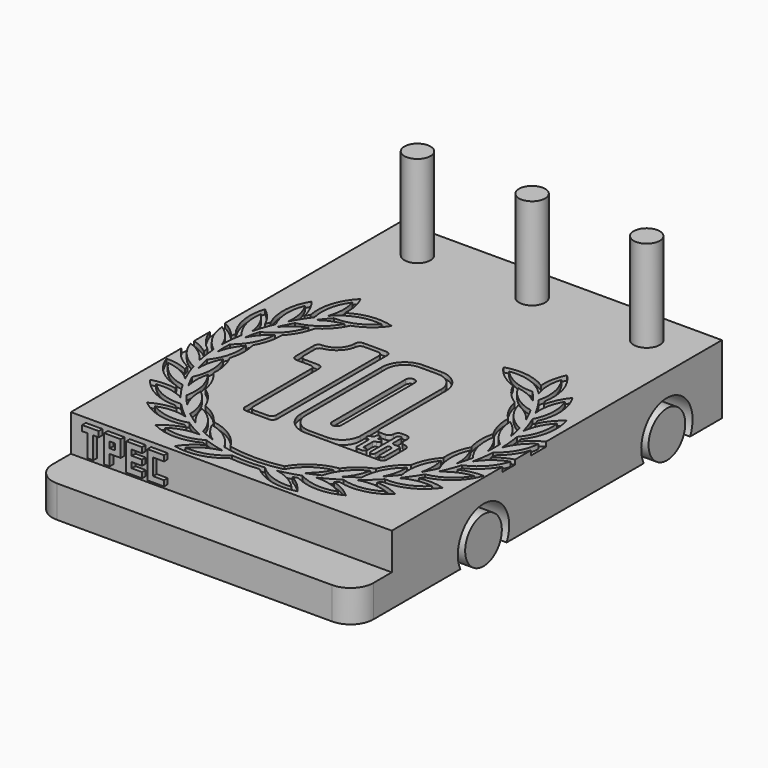
from build123d import *

# Parameters (mm, degrees)
F0_W           = 70
F0_H           = 100
F1_DEPTH       = 15
F2_W           = 70
F2_H           = 10
F3_DEPTH       = 8
F4_R           = 2.85
F5_DEPTH       = 20
F7_R           = 5
F8_DEPTH       = 35
F8_DEPTH_BACK  = 35
F10_DEPTH      = 25
F10_DEPTH_BACK = 25
F11_R          = 7
F11_R_2        = 5
F12_DEPTH      = 10
F13_R          = 7
F13_R_2        = 5
F14_DEPTH      = 10
F15_R          = 5
F16_W          = 1.2
F16_H          = 1.3280942544
F17_DEPTH      = 1
F19_DEPTH      = 1
F21_DEPTH      = 1
F23_DEPTH      = 1
F24_R          = 0.99999
F25_R          = 0.49999


# Not quite as in the source:
# - a fillet or chamfer is up to 0.001 mm smaller than in the source, because OpenCascade refuses the exact size
# - ends of sketch curves that miss each other by under 0.0002 mm in the source are joined


with BuildPart() as f1:
    # F0 (on Top) → F1 (new body)
    with BuildSketch(Plane.XY):
        Rectangle(F0_W, F0_H)
    extrude(amount=F1_DEPTH)

    # F2 (on face) → F3 (cut)
    with BuildSketch(Plane.XY.offset(15)):
        with Locations((0, -45)):
            Rectangle(F2_W, F2_H)
    extrude(amount=-F3_DEPTH, mode=Mode.SUBTRACT)

    # F4 (on face) → F5 (join)
    with BuildSketch(Plane.XY.offset(15)):
        with Locations((0, 42)):
            Circle(F4_R)
        with Locations((-25, 42)):
            Circle(F4_R)
        with Locations((25, 42)):
            Circle(F4_R)
    extrude(amount=F5_DEPTH)

    # F7 (on Right) → F8 (join, two sides)
    with BuildSketch(Plane.YZ) as f8_sk:
        with Locations((-15, 3)):
            Circle(F7_R)
        with Locations((35, 3)):
            Circle(F7_R)
    extrude(amount=F8_DEPTH)
    extrude(f8_sk.sketch, amount=-F8_DEPTH_BACK)

    # F9 (on Right) → F10 (cut, two sides)
    with BuildSketch(Plane.YZ) as f10_sk:
        with BuildLine():
            Line((-11, 0), (-19, 0))
            ThreePointArc((-19, 0), (-15, -2), (-11, 0))
        make_face()
        with BuildLine():
            Line((39, 0), (31, 0))
            ThreePointArc((31, 0), (35, -2), (39, 0))
        make_face()
    extrude(amount=-F10_DEPTH, mode=Mode.SUBTRACT)
    extrude(f10_sk.sketch, amount=F10_DEPTH_BACK, mode=Mode.SUBTRACT)

    # F11 (on face) → F12 (cut)
    with BuildSketch(Plane.YZ.offset(35)):
        with Locations((-15, 3)):
            Circle(F11_R)
        with Locations((-15, 3)):
            Circle(F11_R_2, mode=Mode.SUBTRACT)
        with Locations((35, 3)):
            Circle(F11_R)
        with Locations((35, 3)):
            Circle(F11_R_2, mode=Mode.SUBTRACT)
    extrude(amount=-F12_DEPTH, mode=Mode.SUBTRACT)

    # F13 (on face) → F14 (cut)
    with BuildSketch(Plane(origin=(-35, 0, 0), x_dir=(0, -1, 0), z_dir=(-1, 0, 0))):
        with Locations((15, 3)):
            Circle(F13_R)
        with Locations((15, 3)):
            Circle(F13_R_2, mode=Mode.SUBTRACT)
        with Locations((-35, 3)):
            Circle(F13_R)
        with Locations((-35, 3)):
            Circle(F13_R_2, mode=Mode.SUBTRACT)
    extrude(amount=-F14_DEPTH, mode=Mode.SUBTRACT)

    # F15
    f15_edges = [f1.edges().sort_by_distance(p)[0] for p in [
        (35, -50, 3.5),
        (-35, -50, 3.5),
    ]]
    fillet(f15_edges, radius=F15_R)

    # F16 (on face) → F17 (join)
    with BuildSketch(Plane.XZ.offset(40)):
        Polygon((-28.1147292094, 14), (-31.7147292094, 14), (-31.7147292094, 12.8), (-30.5147292094, 12.8), (-30.5147292094, 8), (-29.3147292094, 8), (-29.3147292094, 12.8), (-28.1147292094, 12.8), align=None)
        Polygon((-23.3147292094, 14), (-26.9147292094, 14), (-26.9147292094, 8), (-25.7147292094, 8), (-25.7147292094, 10.4), (-23.3147292094, 10.4), align=None)
        with Locations((-25.1147292094, 12.1359528728)):
            Rectangle(F16_W, F16_H, mode=Mode.SUBTRACT)
        Polygon((-18.6747292094, 14), (-22.1147292094, 14), (-22.1147292094, 8), (-18.6747292094, 8), (-18.6747292094, 9.2), (-20.9147292094, 9.2), (-20.9147292094, 10.4), (-18.6747292094, 10.4), (-18.6747292094, 11.6), (-20.9147292094, 11.6), (-20.9147292094, 12.8), (-18.6747292094, 12.8), align=None)
        Polygon((-13.8747292094, 12.8), (-13.8747292094, 14), (-17.4747292094, 14), (-17.4747292094, 8), (-13.8747292094, 8), (-13.8747292094, 9.2), (-16.2747292094, 9.2), (-16.2747292094, 12.8), align=None)
    extrude(amount=F17_DEPTH)

    # F18 (on face) → F19 (cut)
    with BuildSketch(Plane.XY.offset(15)):
        with BuildLine():
            ThreePointArc((21.3887258181, 17.7264092206), (16.9142472373, 19.3626016034), (12.1676058235, 18.953359167))
            ThreePointArc((12.1676058235, 18.953359167), (14.591215486, 16.340180418), (17.7231115659, 14.6390590482))
            ThreePointArc((17.7231115659, 14.6390590482), (19.4200221668, 12.0422463003), (21.7744615029, 10.0224548638))
            ThreePointArc((21.7744615029, 10.0224548638), (22.8267654259, 7.1043050239), (24.6519445841, 4.5959862493))
            ThreePointArc((24.6519445841, 4.5959862493), (25.0029118524, 1.5138175305), (26.2004349519, -1.3478044677))
            ThreePointArc((26.2004349519, -1.3478044677), (25.8311448292, -4.427831552), (26.3364530897, -7.4884859913))
            ThreePointArc((26.3364530897, -7.4884859913), (25.2668141021, -10.4003263836), (25.0526662245, -13.4950125909))
            ThreePointArc((25.0526662245, -13.4950125909), (23.3403428867, -16.0816882221), (22.4182836385, -19.0435708628))
            ThreePointArc((22.4182836385, -19.0435708628), (20.1555877448, -21.1656333801), (18.5753255788, -23.8350365945))
            ThreePointArc((18.5753255788, -23.8350365945), (15.8842396506, -25.3780850583), (13.7309669091, -27.6111006282))
            ThreePointArc((13.7309669091, -27.6111006282), (9.2041132945, -29.3610412569), (5.8709446294, -32.888743413))
            ThreePointArc((5.8709446294, -32.888743413), (0, -33.5), (-5.8709446294, -32.888743413))
            ThreePointArc((-5.8709446294, -32.888743413), (-9.2041132945, -29.3610412569), (-13.7309669091, -27.6111006282))
            ThreePointArc((-13.7309669091, -27.6111006282), (-15.8842396506, -25.3780850583), (-18.5753255788, -23.8350365945))
            ThreePointArc((-18.5753255788, -23.8350365945), (-20.1555877448, -21.1656333801), (-22.4182836385, -19.0435708628))
            ThreePointArc((-22.4182836385, -19.0435708628), (-23.3403428867, -16.0816882221), (-25.0526662245, -13.4950125909))
            ThreePointArc((-25.0526662245, -13.4950125909), (-25.2668141021, -10.4003263836), (-26.3364530897, -7.4884859913))
            ThreePointArc((-26.3364530897, -7.4884859913), (-25.8311448292, -4.427831552), (-26.2004349519, -1.3478044677))
            ThreePointArc((-26.2004349519, -1.3478044677), (-25.0029118524, 1.5138175305), (-24.6519445841, 4.5959862493))
            ThreePointArc((-24.6519445841, 4.5959862493), (-22.8267654259, 7.1043050239), (-21.7744615029, 10.0224548638))
            ThreePointArc((-21.7744615029, 10.0224548638), (-19.4200221668, 12.0422463003), (-17.7231115659, 14.6390590482))
            ThreePointArc((-17.7231115659, 14.6390590482), (-14.591215486, 16.340180418), (-12.1676058235, 18.953359167))
            ThreePointArc((-12.1676058235, 18.953359167), (-16.9142472373, 19.3626016034), (-21.3887258181, 17.7264092206))
            ThreePointArc((-21.3887258181, 17.7264092206), (-21.5697046499, 20.6456209174), (-22.5135920697, 23.4139465498))
            ThreePointArc((-22.5135920697, 23.4139465498), (-25.2629047542, 18.8188140189), (-25.5168178808, 13.4700299198))
            ThreePointArc((-25.5168178808, 13.4700299198), (-25.8263883801, 13.0346240116), (-26.1285301404, 12.5940305986))
            ThreePointArc((-26.1285301404, 12.5940305986), (-26.9914700696, 15.1700718344), (-28.4594423065, 17.4560533046))
            ThreePointArc((-28.4594423065, 17.4560533046), (-30.074936422, 12.350748027), (-29.088490785, 7.0875846987))
            ThreePointArc((-29.088490785, 7.0875846987), (-29.2893052588, 6.5925233429), (-29.4816949152, 6.0941274973))
            ThreePointArc((-29.4816949152, 6.0941274973), (-30.9154501797, 8.401723565), (-32.8710366422, 10.2875484131))
            ThreePointArc((-32.8710366422, 10.2875484131), (-33.2656204828, 4.9472987179), (-31.0919956218, 0.0534946578))
            ThreePointArc((-31.0919956218, 0.0534946578), (-31.1732281098, -0.4745332598), (-31.2454938862, -1.0038628891))
            ThreePointArc((-31.2454938862, -1.0038628891), (-32.9521784804, 0.735711305), (-35, 2.0568160339))
            Line((-35, 2.0568160339), (-35, -2.1009931114))
            ThreePointArc((-35, -2.1009931114), (-33.5847749975, -4.9377165589), (-31.4193229266, -7.2530305881))
            ThreePointArc((-31.4193229266, -7.2530305881), (-31.3765941644, -7.7855589458), (-31.3248401941, -8.3172860614))
            ThreePointArc((-31.3248401941, -8.3172860614), (-33.0705923516, -7.1776978407), (-35, -6.38795229))
            Line((-35, -6.38795229), (-35, -9.7772099505))
            ThreePointArc((-35, -9.7772099505), (-32.8954370333, -12.4993428364), (-30.0528264, -14.4380943719))
            ThreePointArc((-30.0528264, -14.4380943719), (-29.8884399062, -14.9464144281), (-29.7154562591, -15.4518734835))
            ThreePointArc((-29.7154562591, -15.4518734835), (-32.2970706727, -14.6057524582), (-35.0073216617, -14.4181535604))
            ThreePointArc((-35.0073216617, -14.4181535604), (-31.8769440834, -18.762655768), (-27.0661742232, -21.1143480451))
            ThreePointArc((-27.0661742232, -21.1143480451), (-26.7889921162, -21.571056134), (-26.5041043855, -22.0229977008))
            ThreePointArc((-26.5041043855, -22.0229977008), (-29.2112599855, -21.7950452331), (-31.8917190916, -22.2375299796))
            ThreePointArc((-31.8917190916, -22.2375299796), (-27.8438100865, -25.743010817), (-22.6203775882, -26.9218730442))
            ThreePointArc((-22.6203775882, -26.9218730442), (-22.2453428272, -27.3023479145), (-21.8639093842, -27.6764077058))
            ThreePointArc((-21.8639093842, -27.6764077058), (-24.5506627115, -28.0789127723), (-27.0568256903, -29.1276266959))
            ThreePointArc((-27.0568256903, -29.1276266959), (-22.3096090807, -31.6051047837), (-16.9551105424, -31.5475841932))
            ThreePointArc((-16.9551105424, -31.5475841932), (-16.5024413484, -31.8313143462), (-16.0450253688, -32.1073267018))
            ThreePointArc((-16.0450253688, -32.1073267018), (-18.566532856, -33.1185901502), (-20.7632918127, -34.7169968119))
            ThreePointArc((-20.7632918127, -34.7169968119), (-15.5726912747, -36.0329106651), (-10.3757890986, -34.7421082068))
            ThreePointArc((-10.3757890986, -34.7421082068), (-9.869888985, -34.9137976764), (-9.3611498826, -35.0768826988))
            ThreePointArc((-9.3611498826, -35.0768826988), (-11.5814764084, -36.6423870548), (-13.3504034991, -38.7043159377))
            ThreePointArc((-13.3504034991, -38.7043159377), (-7.9962456512, -38.7877243), (-3.2371061788, -36.3332274684))
            ThreePointArc((-3.2371061788, -36.3332274684), (0, -36.5), (3.2371061788, -36.3332274684))
            ThreePointArc((3.2371061788, -36.3332274684), (7.9962456512, -38.7877243), (13.3504034991, -38.7043159377))
            ThreePointArc((13.3504034991, -38.7043159377), (11.5814764084, -36.6423870548), (9.3611498826, -35.0768826988))
            ThreePointArc((9.3611498826, -35.0768826988), (9.869888985, -34.9137976764), (10.3757890986, -34.7421082068))
            ThreePointArc((10.3757890986, -34.7421082068), (15.5726912747, -36.0329106651), (20.7632918127, -34.7169968119))
            ThreePointArc((20.7632918127, -34.7169968119), (18.566532856, -33.1185901502), (16.0450253688, -32.1073267018))
            ThreePointArc((16.0450253688, -32.1073267018), (16.5024413484, -31.8313143462), (16.9551105424, -31.5475841932))
            ThreePointArc((16.9551105424, -31.5475841932), (22.3096090807, -31.6051047837), (27.0568256903, -29.1276266959))
            ThreePointArc((27.0568256903, -29.1276266959), (24.5506627115, -28.0789127723), (21.8639093842, -27.6764077058))
            ThreePointArc((21.8639093842, -27.6764077058), (22.2453428272, -27.3023479145), (22.6203775882, -26.9218730442))
            ThreePointArc((22.6203775882, -26.9218730442), (27.8438100865, -25.743010817), (31.8917190916, -22.2375299796))
            ThreePointArc((31.8917190916, -22.2375299796), (29.2112599855, -21.7950452331), (26.5041043855, -22.0229977008))
            ThreePointArc((26.5041043855, -22.0229977008), (26.7889921162, -21.571056134), (27.0661742232, -21.1143480451))
            ThreePointArc((27.0661742232, -21.1143480451), (31.8769440834, -18.762655768), (35.0073216617, -14.4181535604))
            ThreePointArc((35.0073216617, -14.4181535604), (32.2970706727, -14.6057524582), (29.7154562591, -15.4518734835))
            ThreePointArc((29.7154562591, -15.4518734835), (29.8884399062, -14.9464144281), (30.0528264, -14.4380943719))
            ThreePointArc((30.0528264, -14.4380943719), (32.8954370333, -12.4993428364), (35, -9.7772099505))
            Line((35, -9.7772099505), (35, -6.38795229))
            ThreePointArc((35, -6.38795229), (33.0705923516, -7.1776978407), (31.3248401941, -8.3172860614))
            ThreePointArc((31.3248401941, -8.3172860614), (31.3765941644, -7.7855589458), (31.4193229266, -7.2530305881))
            ThreePointArc((31.4193229266, -7.2530305881), (33.5847749975, -4.9377165589), (35, -2.1009931114))
            Line((35, -2.1009931114), (35, 2.0568160339))
            ThreePointArc((35, 2.0568160339), (32.9521784804, 0.735711305), (31.2454938862, -1.0038628891))
            ThreePointArc((31.2454938862, -1.0038628891), (31.1732281098, -0.4745332598), (31.0919956218, 0.0534946578))
            ThreePointArc((31.0919956218, 0.0534946578), (33.2656204828, 4.9472987179), (32.8710366422, 10.2875484131))
            ThreePointArc((32.8710366422, 10.2875484131), (30.9154501797, 8.401723565), (29.4816949152, 6.0941274973))
            ThreePointArc((29.4816949152, 6.0941274973), (29.2893052588, 6.5925233429), (29.088490785, 7.0875846987))
            ThreePointArc((29.088490785, 7.0875846987), (30.074936422, 12.350748027), (28.4594423065, 17.4560533046))
            ThreePointArc((28.4594423065, 17.4560533046), (26.9914700696, 15.1700718344), (26.1285301404, 12.5940305986))
            ThreePointArc((26.1285301404, 12.5940305986), (25.8263883801, 13.0346240116), (25.5168178808, 13.4700299198))
            ThreePointArc((25.5168178808, 13.4700299198), (25.2629047542, 18.8188140189), (22.5135920697, 23.4139465498))
            ThreePointArc((22.5135920697, 23.4139465498), (21.5697046499, 20.6456209174), (21.3887258181, 17.7264092206))
        make_face()
        with BuildLine():
            ThreePointArc((10.4677081127, -33.6474621366), (8.2010145811, -34.3767486261), (5.884336883, -34.926987477))
            ThreePointArc((5.884336883, -34.926987477), (8.9752410442, -36.0049666829), (11.5524222343, -38.0233484147))
            ThreePointArc((11.5524222343, -38.0233484147), (7.2635603893, -37.5374744103), (3.5789902606, -35.2892857082))
            ThreePointArc((3.5789902606, -35.2892857082), (0, -35.5), (-3.5789902606, -35.2892857082))
            ThreePointArc((-3.5789902606, -35.2892857082), (-7.2635603893, -37.5374744103), (-11.5524222343, -38.0233484147))
            ThreePointArc((-11.5524222343, -38.0233484147), (-8.9752410442, -36.0049666829), (-5.884336883, -34.926987477))
            ThreePointArc((-5.884336883, -34.926987477), (-8.2010145811, -34.3767486261), (-10.4677081127, -33.6474621366))
            ThreePointArc((-10.4677081127, -33.6474621366), (-14.5714281718, -34.9853302727), (-18.8567334473, -34.4690278716))
            ThreePointArc((-18.8567334473, -34.4690278716), (-15.8835496492, -33.0993907648), (-12.6273620965, -32.7632801824))
            ThreePointArc((-12.6273620965, -32.7632801824), (-14.7546996357, -31.6936104463), (-16.792109111, -30.4612464661))
            ThreePointArc((-16.792109111, -30.4612464661), (-21.09374649, -30.8166692186), (-25.1444732793, -29.3260244081))
            ThreePointArc((-25.1444732793, -29.3260244081), (-21.9355719813, -28.6789694172), (-18.6896429508, -29.1028472669))
            ThreePointArc((-18.6896429508, -29.1028472669), (-20.5129550138, -27.5714128181), (-22.2112431606, -25.9024084081))
            ThreePointArc((-22.2112431606, -25.9024084081), (-26.4788954749, -25.2562248446), (-30.0766680485, -22.8715986722))
            ThreePointArc((-30.0766680485, -22.8715986722), (-26.80504195, -22.9820086994), (-23.7443603161, -24.1430236164))
            ThreePointArc((-23.7443603161, -24.1430236164), (-25.1653516775, -22.2323844823), (-26.4329633423, -20.2167161026))
            ThreePointArc((-26.4329633423, -20.2167161026), (-30.436560351, -18.6037621462), (-33.3874218581, -15.4537104261))
            ThreePointArc((-33.3874218581, -15.4537104261), (-30.2294451691, -16.315633238), (-27.5190130707, -18.1511946078))
            ThreePointArc((-27.5190130707, -18.1511946078), (-28.4610777185, -15.9643538388), (-29.2296756283, -13.7106866932))
            ThreePointArc((-29.2296756283, -13.7106866932), (-32.7533823803, -11.2179171092), (-34.8982511133, -7.472259945))
            ThreePointArc((-34.8982511133, -7.472259945), (-32.0241711744, -9.0392290599), (-29.8101087077, -11.4503812939))
            ThreePointArc((-29.8101087077, -11.4503812939), (-30.2224596928, -9.1052320417), (-30.4506085353, -6.7350619095))
            ThreePointArc((-30.4506085353, -6.7350619095), (-33.3044610876, -3.4968625514), (-34.5277066179, 0.6424707097))
            ThreePointArc((-34.5277066179, 0.6424707097), (-32.0924658226, -1.5450689977), (-30.4941336681, -4.4018262547))
            ThreePointArc((-30.4941336681, -4.4018262547), (-30.3545410423, -2.0247961227), (-30.0299412544, 0.3341005108))
            ThreePointArc((-30.0299412544, 0.3341005108), (-32.0600876772, 4.1431574775), (-32.2957645216, 8.4530143079))
            ThreePointArc((-32.2957645216, 8.4530143079), (-30.4306473315, 5.76283484), (-29.5342119894, 2.614481083))
            ThreePointArc((-29.5342119894, 2.614481083), (-28.8502012272, 4.8952457852), (-27.9903520674, 7.1157001919))
            ThreePointArc((-27.9903520674, 7.1157001919), (-29.0873466416, 11.2902675201), (-28.3227494004, 15.5383024226))
            ThreePointArc((-28.3227494004, 15.5383024226), (-27.1283047661, 12.4905114656), (-26.9820932977, 9.2202897745))
            ThreePointArc((-26.9820932977, 9.2202897745), (-25.7905395964, 11.2818324315), (-24.4417957555, 13.2441393397))
            ThreePointArc((-24.4417957555, 13.2441393397), (-24.5464992196, 17.5591650242), (-22.8228475281, 21.5163653375))
            ThreePointArc((-22.8228475281, 21.5163653375), (-22.3634682688, 18.2752700908), (-22.9753629723, 15.0594789636))
            ThreePointArc((-22.9753629723, 15.0594789636), (-18.8621153758, 17.8634174598), (-13.9066335748, 18.3367851817))
            ThreePointArc((-13.9066335748, 18.3367851817), (-17.4158522627, 15.8293894225), (-21.6546703391, 15.0331039159))
            ThreePointArc((-21.6546703391, 15.0331039159), (-22.7940667976, 13.7264657324), (-23.8547408227, 12.3551531333))
            ThreePointArc((-23.8547408227, 12.3551531333), (-21.5313635149, 13.7668770297), (-18.913611502, 14.5006487059))
            ThreePointArc((-18.913611502, 14.5006487059), (-21.7499934897, 11.2515586006), (-25.6909176008, 9.4991983512))
            ThreePointArc((-25.6909176008, 9.4991983512), (-26.4982699779, 7.9650178627), (-27.2141069483, 6.3860609083))
            ThreePointArc((-27.2141069483, 6.3860609083), (-25.2789225121, 8.2955392853), (-22.9009517375, 9.6132272109))
            ThreePointArc((-22.9009517375, 9.6132272109), (-24.9115869379, 5.7976020479), (-28.3421608448, 3.1836372505))
            ThreePointArc((-28.3421608448, 3.1836372505), (-28.7739445648, 1.5046225242), (-29.1063535241, -0.1968568074))
            ThreePointArc((-29.1063535241, -0.1968568074), (-27.6636882534, 2.1074355766), (-25.6536957372, 3.9380028544))
            ThreePointArc((-25.6536957372, 3.9380028544), (-26.7301902861, -0.2384560259), (-29.4654708615, -3.5731058527))
            ThreePointArc((-29.4654708615, -3.5731058527), (-29.4984083524, -5.3064386983), (-29.4294690476, -7.0387132159))
            ThreePointArc((-29.4294690476, -7.0387132159), (-28.5570974006, -4.4638318237), (-27.0234423594, -2.2190715495))
            ThreePointArc((-27.0234423594, -2.2190715495), (-27.1077621572, -6.5312101679), (-29.0002897173, -10.4067731886))
            ThreePointArc((-29.0002897173, -10.4067731886), (-28.6326053103, -12.1009797312), (-28.1660342772, -13.7706620672))
            ThreePointArc((-28.1660342772, -13.7706620672), (-27.9109860351, -11.0640041892), (-26.9363482093, -8.526066526))
            ThreePointArc((-26.9363482093, -8.526066526), (-26.0239475538, -12.7414163735), (-26.9716954479, -16.9489599825))
            ThreePointArc((-26.9716954479, -16.9489599825), (-26.2232111047, -18.5127051088), (-25.3841613084, -20.0297822563))
            ThreePointArc((-25.3841613084, -20.0297822563), (-25.760186188, -17.3372645193), (-25.3971085551, -14.6429703433))
            ThreePointArc((-25.3971085551, -14.6429703433), (-23.5371752017, -18.5342808185), (-23.4890500956, -22.8469752509))
            ThreePointArc((-23.4890500956, -22.8469752509), (-22.4001168008, -24.1959570564), (-21.233821633, -25.4786429936))
            ThreePointArc((-21.233821633, -25.4786429936), (-22.2206480357, -22.9454197257), (-22.4887042048, -20.2400191335))
            ThreePointArc((-22.4887042048, -20.2400191335), (-19.7815076421, -23.5975086814), (-18.7401039727, -27.782855464))
            ThreePointArc((-18.7401039727, -27.782855464), (-17.3694264021, -28.8443499903), (-15.9387611372, -29.8234947864))
            ThreePointArc((-15.9387611372, -29.8234947864), (-17.4831889962, -27.5861327097), (-18.3679279899, -25.0154745474))
            ThreePointArc((-18.3679279899, -25.0154745474), (-14.9594138853, -27.6581400375), (-12.980873994, -31.4905060418))
            ThreePointArc((-12.980873994, -31.4905060418), (-11.4023457302, -32.2072878444), (-9.7844379029, -32.83010555))
            ThreePointArc((-9.7844379029, -32.83010555), (-11.8032067126, -31.0092214332), (-13.2569320226, -28.7118905477))
            ThreePointArc((-13.2569320226, -28.7118905477), (-9.3308542538, -30.4972651993), (-6.5218417382, -33.7700465822))
            ThreePointArc((-6.5218417382, -33.7700465822), (0, -34.5), (6.5218417382, -33.7700465822))
            ThreePointArc((6.5218417382, -33.7700465822), (9.3308542538, -30.4972651993), (13.2569320226, -28.7118905477))
            ThreePointArc((13.2569320226, -28.7118905477), (11.8032067126, -31.0092214332), (9.7844379029, -32.83010555))
            ThreePointArc((9.7844379029, -32.83010555), (11.4023457302, -32.2072878444), (12.980873994, -31.4905060418))
            ThreePointArc((12.980873994, -31.4905060418), (14.9594138853, -27.6581400375), (18.3679279899, -25.0154745474))
            ThreePointArc((18.3679279899, -25.0154745474), (17.4831889962, -27.5861327097), (15.9387611372, -29.8234947864))
            ThreePointArc((15.9387611372, -29.8234947864), (17.3694264021, -28.8443499903), (18.7401039727, -27.782855464))
            ThreePointArc((18.7401039727, -27.782855464), (19.7815076421, -23.5975086814), (22.4887042048, -20.2400191335))
            ThreePointArc((22.4887042048, -20.2400191335), (22.2206480357, -22.9454197257), (21.233821633, -25.4786429936))
            ThreePointArc((21.233821633, -25.4786429936), (22.4001168008, -24.1959570564), (23.4890500956, -22.8469752509))
            ThreePointArc((23.4890500956, -22.8469752509), (23.5371752017, -18.5342808185), (25.3971085551, -14.6429703433))
            ThreePointArc((25.3971085551, -14.6429703433), (25.760186188, -17.3372645193), (25.3841613084, -20.0297822563))
            ThreePointArc((25.3841613084, -20.0297822563), (26.2232111047, -18.5127051088), (26.9716954479, -16.9489599825))
            ThreePointArc((26.9716954479, -16.9489599825), (26.0239475538, -12.7414163735), (26.9363482093, -8.526066526))
            ThreePointArc((26.9363482093, -8.526066526), (27.9109860351, -11.0640041892), (28.1660342772, -13.7706620672))
            ThreePointArc((28.1660342772, -13.7706620672), (28.6326053103, -12.1009797312), (29.0002897173, -10.4067731886))
            ThreePointArc((29.0002897173, -10.4067731886), (27.1077621572, -6.5312101679), (27.0234423594, -2.2190715495))
            ThreePointArc((27.0234423594, -2.2190715495), (28.5570974006, -4.4638318237), (29.4294690476, -7.0387132159))
            ThreePointArc((29.4294690476, -7.0387132159), (29.4984083524, -5.3064386983), (29.4654708615, -3.5731058527))
            ThreePointArc((29.4654708615, -3.5731058527), (26.7301902861, -0.2384560259), (25.6536957372, 3.9380028544))
            ThreePointArc((25.6536957372, 3.9380028544), (27.6636882534, 2.1074355766), (29.1063535241, -0.1968568074))
            ThreePointArc((29.1063535241, -0.1968568074), (28.7739445648, 1.5046225242), (28.3421608448, 3.1836372505))
            ThreePointArc((28.3421608448, 3.1836372505), (24.9115869379, 5.7976020479), (22.9009517375, 9.6132272109))
            ThreePointArc((22.9009517375, 9.6132272109), (25.2789225121, 8.2955392853), (27.2141069483, 6.3860609083))
            ThreePointArc((27.2141069483, 6.3860609083), (26.4982699779, 7.9650178627), (25.6909176008, 9.4991983512))
            ThreePointArc((25.6909176008, 9.4991983512), (21.7499934897, 11.2515586006), (18.913611502, 14.5006487059))
            ThreePointArc((18.913611502, 14.5006487059), (21.5313635149, 13.7668770297), (23.8547408227, 12.3551531333))
            ThreePointArc((23.8547408227, 12.3551531333), (22.7940667976, 13.7264657324), (21.6546703391, 15.0331039159))
            ThreePointArc((21.6546703391, 15.0331039159), (17.4158522627, 15.8293894225), (13.9066335748, 18.3367851817))
            ThreePointArc((13.9066335748, 18.3367851817), (18.8621153758, 17.8634174598), (22.9753629723, 15.0594789636))
            ThreePointArc((22.9753629723, 15.0594789636), (22.3634682688, 18.2752700908), (22.8228475281, 21.5163653375))
            ThreePointArc((22.8228475281, 21.5163653375), (24.5464992196, 17.5591650242), (24.4417957555, 13.2441393397))
            ThreePointArc((24.4417957555, 13.2441393397), (25.7905395964, 11.2818324315), (26.9820932977, 9.2202897745))
            ThreePointArc((26.9820932977, 9.2202897745), (27.1283047661, 12.4905114656), (28.3227494004, 15.5383024226))
            ThreePointArc((28.3227494004, 15.5383024226), (29.0873466416, 11.2902675201), (27.9903520674, 7.1157001919))
            ThreePointArc((27.9903520674, 7.1157001919), (28.8502012272, 4.8952457852), (29.5342119894, 2.614481083))
            ThreePointArc((29.5342119894, 2.614481083), (30.4306473315, 5.76283484), (32.2957645216, 8.4530143079))
            ThreePointArc((32.2957645216, 8.4530143079), (32.0600876772, 4.1431574775), (30.0299412544, 0.3341005108))
            ThreePointArc((30.0299412544, 0.3341005108), (30.3545410423, -2.0247961227), (30.4941336681, -4.4018262547))
            ThreePointArc((30.4941336681, -4.4018262547), (32.0924658226, -1.5450689977), (34.5277066179, 0.6424707097))
            ThreePointArc((34.5277066179, 0.6424707097), (33.3044610876, -3.4968625514), (30.4506085353, -6.7350619095))
            ThreePointArc((30.4506085353, -6.7350619095), (30.2224596928, -9.1052320417), (29.8101087077, -11.4503812939))
            ThreePointArc((29.8101087077, -11.4503812939), (32.0241711744, -9.0392290599), (34.8982511133, -7.472259945))
            ThreePointArc((34.8982511133, -7.472259945), (32.7533823803, -11.2179171092), (29.2296756283, -13.7106866932))
            ThreePointArc((29.2296756283, -13.7106866932), (28.4610777185, -15.9643538388), (27.5190130707, -18.1511946078))
            ThreePointArc((27.5190130707, -18.1511946078), (30.2294451691, -16.315633238), (33.3874218581, -15.4537104261))
            ThreePointArc((33.3874218581, -15.4537104261), (30.436560351, -18.6037621462), (26.4329633423, -20.2167161026))
            ThreePointArc((26.4329633423, -20.2167161026), (25.1653516775, -22.2323844823), (23.7443603161, -24.1430236164))
            ThreePointArc((23.7443603161, -24.1430236164), (26.80504195, -22.9820086994), (30.0766680485, -22.8715986722))
            ThreePointArc((30.0766680485, -22.8715986722), (26.4788954749, -25.2562248446), (22.2112431606, -25.9024084081))
            ThreePointArc((22.2112431606, -25.9024084081), (20.5129550138, -27.5714128181), (18.6896429508, -29.1028472669))
            ThreePointArc((18.6896429508, -29.1028472669), (21.9355719813, -28.6789694172), (25.1444732793, -29.3260244081))
            ThreePointArc((25.1444732793, -29.3260244081), (21.09374649, -30.8166692186), (16.792109111, -30.4612464661))
            ThreePointArc((16.792109111, -30.4612464661), (14.7546996357, -31.6936104463), (12.6273620965, -32.7632801824))
            ThreePointArc((12.6273620965, -32.7632801824), (15.8835496492, -33.0993907648), (18.8567334473, -34.4690278716))
            ThreePointArc((18.8567334473, -34.4690278716), (14.5714281718, -34.9853302727), (10.4677081127, -33.6474621366))
        make_face(mode=Mode.SUBTRACT)
    extrude(amount=-F19_DEPTH, mode=Mode.SUBTRACT)

    # F20 (on face) → F21 (cut)
    with BuildSketch(Plane.XY.offset(15)):
        with BuildLine():
            Line((-6, -21), (-6, 11))
            Line((-6, 11), (-13, 11))
            Line((-13, 11), (-13, 10))
            ThreePointArc((-13, 10), (-14.1715728753, 7.1715728753), (-17, 6))
            Line((-17, 6), (-18, 6))
            Line((-18, 6), (-18, 5))
            Line((-18, 5), (-18, -1))
            Line((-18, -1), (-13, -1))
            Line((-13, -1), (-13, -21))
            Line((-13, -21), (-6, -21))
        make_face()
        with BuildLine():
            ThreePointArc((-17, 5), (-13.4644660941, 6.4644660941), (-12, 10))
            Line((-12, 10), (-7, 10))
            Line((-7, 10), (-7, -20))
            Line((-7, -20), (-12, -20))
            Line((-12, -20), (-12, 0))
            Line((-12, 0), (-17, 0))
            Line((-17, 0), (-17, 5))
        make_face(mode=Mode.SUBTRACT)
        with BuildLine():
            Line((5.0000001751, 11), (1.0000004899, 11))
            ThreePointArc((1.0000004899, 11), (-2.5355337327, 9.5355340791), (-4, 6))
            Line((-4, 6), (-4, -16))
            ThreePointArc((-4, -16), (-2.5355339059, -19.5355339059), (1, -21))
            Line((1, -21), (5, -21))
            Line((5, -21), (10, -21))
            Line((10, -21), (18, -21))
            Line((18, -21), (18, -14))
            Line((18, -14), (16, -14))
            Line((16, -14), (16, -11))
            Line((16, -11), (13, -11))
            Line((13, -11), (13, -13))
            Line((13, -13), (10, -13))
            Line((10, -13), (10, 6))
            ThreePointArc((10, 6), (8.5355339678, 9.535533844), (5.0000001751, 11))
        make_face()
        Polygon((11, -15), (11, -14), (12, -14), (12, -15), (13, -15), (13, -16), (12, -16), (12, -19), (13, -19), (13, -20), (12, -20), (11, -20), (11, -16), (10, -16), (10, -15), align=None, mode=Mode.SUBTRACT)
        Polygon((14, -17), (14, -14), (14, -12), (15, -12), (15, -15), (17, -15), (17, -20), (16, -20), (16, -16), (15, -16), (15, -20), (14, -20), align=None, mode=Mode.SUBTRACT)
        with BuildLine():
            ThreePointArc((-3, 6), (-1.8284271247, 8.8284271247), (1, 10))
            Line((1, 10), (5, 10))
            ThreePointArc((5, 10), (7.8284271247, 8.8284271247), (9, 6))
            Line((9, 6), (9, -16))
            ThreePointArc((9, -16), (7.8284271247, -18.8284271247), (5, -20))
            Line((5, -20), (1, -20))
            ThreePointArc((1, -20), (-1.8284271247, -18.8284271247), (-3, -16))
            Line((-3, -16), (-3, 6))
        make_face(mode=Mode.SUBTRACT)
        with BuildLine():
            ThreePointArc((3, 6), (2.2928932188, 5.7071067812), (2, 5))
            Line((2, 5), (2, -15))
            ThreePointArc((2, -15), (2.2928932188, -15.7071067812), (3, -16))
            ThreePointArc((3, -16), (3.7071074462, -15.7071067812), (4.000000665, -15))
            Line((4.000000665, -15), (4.000000665, 5))
            ThreePointArc((4.000000665, 5), (3.7071074462, 5.7071067812), (3, 6))
        make_face()
    extrude(amount=-F21_DEPTH, mode=Mode.SUBTRACT)

    # F22 (on face) → F23 (join, through all)
    with BuildSketch(Plane.XY.offset(14)):
        with BuildLine():
            ThreePointArc((27.0661742232, -21.1143480451), (31.8693847915, -18.7690241624), (35, -14.4365163097))
            Line((35, -14.4365163097), (35, -14.4177551427))
            ThreePointArc((35, -14.4177551427), (34.8000652295, -14.408765597), (34.6, -14.4034150522))
            ThreePointArc((34.6, -14.4034150522), (31.723711099, -18.7587136079), (27.0661742232, -21.1143480451))
        make_face()
        with BuildLine():
            ThreePointArc((-35, -14.4365163097), (-31.8693847915, -18.7690241624), (-27.0661742232, -21.1143480451))
            ThreePointArc((-27.0661742232, -21.1143480451), (-31.723711099, -18.7587136079), (-34.6, -14.4034150522))
            ThreePointArc((-34.6, -14.4034150522), (-34.8000652295, -14.408765597), (-35, -14.4177551427))
            Line((-35, -14.4177551427), (-35, -14.4365163097))
        make_face()
    extrude(amount=F23_DEPTH)

    # F24 (radius 1 in the source; OpenCascade refuses exactly that, so slightly less here)
    f24_edges = [f1.edges().sort_by_distance(p)[0] for p in [
        (16, -14, 14.5),
        (13, -13, 14.5),
        (13, -11, 14.5),
        (16, -11, 14.5),
        (18, -14, 14.5),
        (18, -21, 14.5),
        (10, -13, 14.5),
        (-13, 11, 14.5),
        (-6, 11, 14.5),
        (-18, 6, 14.5),
        (-18, -1, 14.5),
        (-13, -1, 14.5),
        (-13, -21, 14.5),
        (-6, -21, 14.5),
        (-12, -20, 14.5),
        (-7, -20, 14.5),
        (-12, 0, 14.5),
        (-17, 0, 14.5),
        (-17, 5, 14.5),
        (-12, 10, 14.5),
        (-7, 10, 14.5),
    ]]
    fillet(f24_edges, radius=F24_R)

    # F25 (radius 0.5 in the source; OpenCascade refuses exactly that, so slightly less here)
    f25_edges = [f1.edges().sort_by_distance(p)[0] for p in [
        (10, -15, 14.5),
        (11, -15, 14.5),
        (11, -14, 14.5),
        (12, -14, 14.5),
        (13, -15, 14.5),
        (13, -19, 14.5),
        (11, -20, 14.5),
        (10, -16, 14.5),
        (11, -16, 14.5),
        (13, -16, 14.5),
        (13, -20, 14.5),
        (12, -16, 14.5),
        (15, -16, 14.5),
        (15, -20, 14.5),
        (14, -20, 14.5),
        (16, -20, 14.5),
        (17, -20, 14.5),
        (17, -15, 14.5),
        (15, -12, 14.5),
        (16, -16, 14.5),
        (15, -15, 14.5),
        (14, -12, 14.5),
    ]]
    fillet(f25_edges, radius=F25_R)


solid = f1.part
